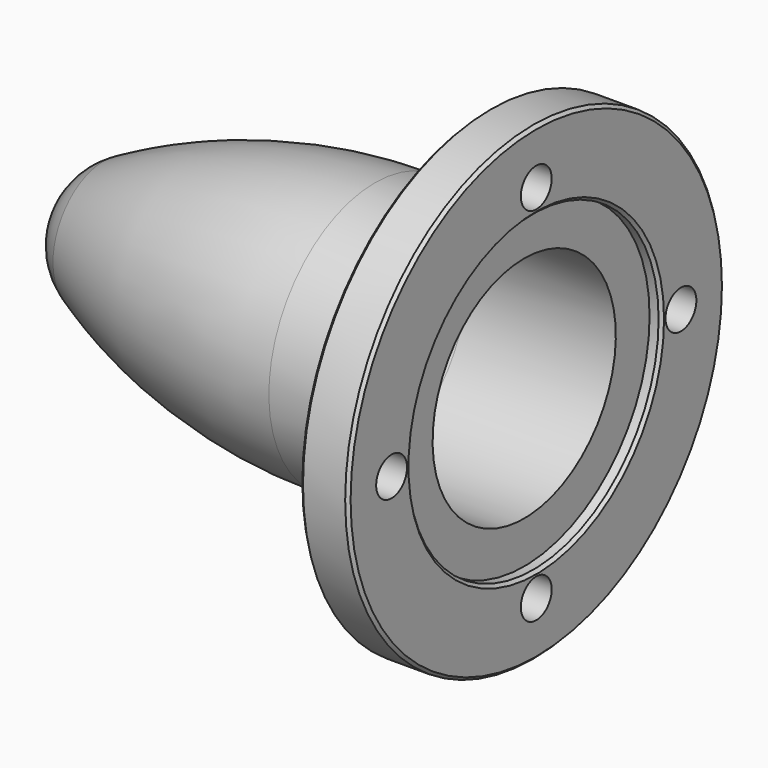
from build123d import *

# Parameters (mm, degrees)
F2_T            = -1.5
F3_R            = 19.5
F3_R_2          = 11
F4_DEPTH        = 4
F5_R            = 13
F6_DEPTH        = 1
F7_SIZE         = 0.25
F9_D            = 3.2
F9_COPIES_COUNT = 4


# Not quite as in the source:
# - a pattern or mirror of a feature is missing from the dataset's text; its kind, count and spacing are read off the source's solid


with BuildPart() as f1:
    # F0 (on Front) → F1 (revolve)
    with BuildSketch(Plane.XZ):
        with BuildLine():
            Line((-39.0004168703, 0), (0, 0))
            Line((0, 0), (0, 11))
            Line((0, 11), (-13.379, 11))
            ThreePointArc((-13.379, 11), (-24.9848227606, 9.544537302), (-35.8718437294, 5.2682926829))
            ThreePointArc((-35.8718437294, 5.2682926829), (-38.1593199105, 3.0636121528), (-39.0004168703, 0))
        make_face()
    revolve(axis=Axis((-19.5002084352, 0, 0), (1, 0, 0)))

    # F2
    f2_openings = [f1.faces().sort_by_distance(p)[0] for p in [
        (0, 0, 0),
    ]]
    offset(amount=F2_T, openings=f2_openings)

    # F3 (on Right) → F4 (join)
    with BuildSketch(Plane.YZ):
        Circle(F3_R)
        Circle(F3_R_2, mode=Mode.SUBTRACT)
    extrude(amount=-F4_DEPTH)

    # F5 (on Right) → F6 (cut)
    with BuildSketch(Plane.YZ):
        Circle(F5_R)
    extrude(amount=-F6_DEPTH, mode=Mode.SUBTRACT)

    # F7
    f7_edges = [f1.edges().sort_by_distance(p)[0] for p in [
        (-4, -19.5, 0),
        (-4, 0, -11),
        (0, -19.5, 0),
        (0, -13, 0),
    ]]
    chamfer(f7_edges, length=F7_SIZE)

    # F9 (through all)
    with Locations(Plane.YZ):
        with Locations((0, 15)):
            f9 = Hole(F9_D / 2)

    # F9_copies: F9 ×4 about axis
    f9_copies_axis = Axis((0, 0, 0), (1, 0, 0))
    for i in range(1, F9_COPIES_COUNT):
        add(f9.rotate(f9_copies_axis, i * 360 / F9_COPIES_COUNT), mode=Mode.SUBTRACT)


solid = f1.part
